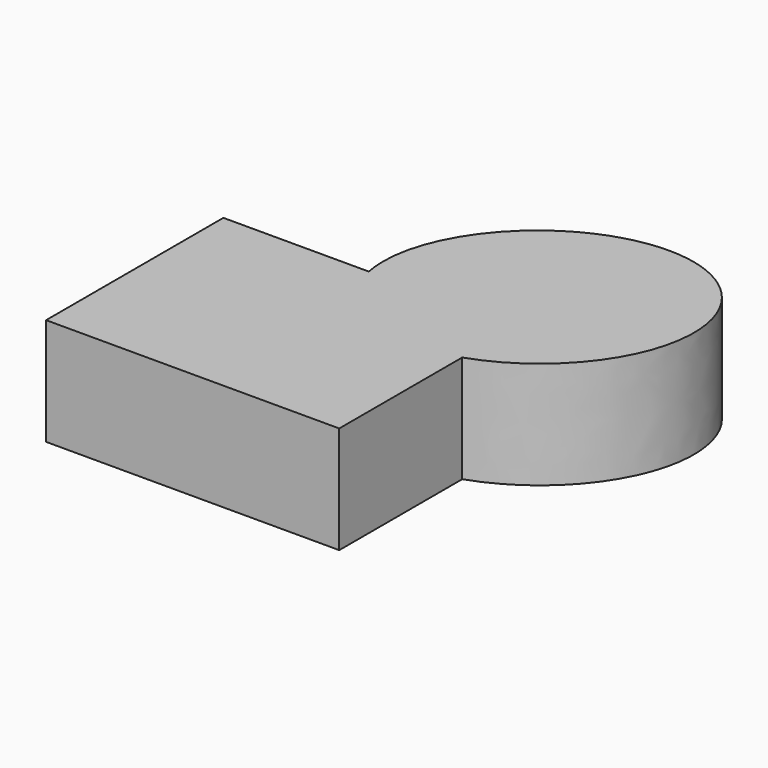
from build123d import *

# Parameters (mm, degrees)
F0_W     = 69.4850608706
F0_H     = 52.5225289166
F4_DEPTH = 25.4
F5_DEPTH = 25.4


# Not quite as in the source:
# - the program builds the solid bodies; features that only make, move or delete a surface that nothing else refers to are left out


with BuildPart() as f4:
    # F0 (on Top) → F4 (new body)
    with BuildSketch(Plane.XY):
        Rectangle(F0_W, F0_H)
    extrude(amount=F4_DEPTH)

    # F3 (on face) → F5 (join)
    with BuildSketch(Plane.XY):
        with BuildLine():
            Line((34.7425304353, 26.2612644583), (34.7425304353, 10.1695671882))
            add(Edge.make_bspline(
                [(34.7425304353, 10.1695671882), (112.2797997443, 36.2054211909), (49.2358666955, 65.1774495788), (-13.8080663534, 94.1494779666), (-0.2734467602, 26.2612644583)],
                knots=[1.1513743417, 1.1513743417, 1.1513743417, 3.5292771676, 3.5292771676, 5.9071799934, 5.9071799934, 5.9071799934], degree=2, weights=[1, 0.3726331435, 1, 0.3726331435, 1]))
            Line((-0.2734467602, 26.2612644583), (34.7425304353, 26.2612644583))
        make_face()
    extrude(amount=F5_DEPTH)


solid = f4.part
